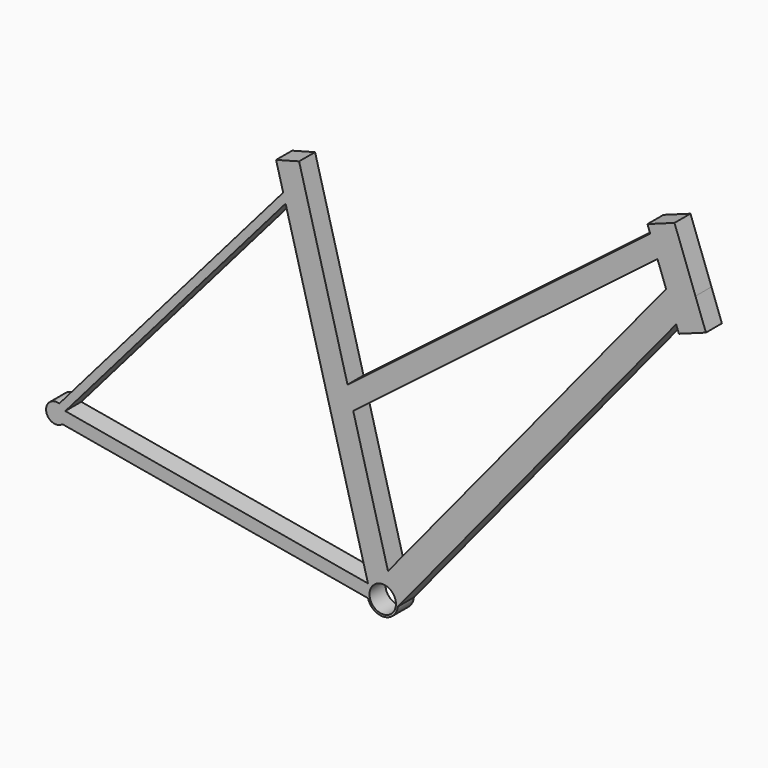
from build123d import *

# Parameters (mm, degrees)
F1_R     = 16.55
F0_DEPTH = 25


with BuildPart() as f0:
    # F1 (on Front) → F0 (new body)
    with BuildSketch(Plane.XZ):
        with BuildLine():
            ThreePointArc((18.9471511403, -1.9768570177), (19.0242704094, -0.9897653202), (19.05, 0))
            ThreePointArc((19.05, 0), (17.0081092666, 8.5806013294), (11.3201607165, 15.3217643028))
            ThreePointArc((11.3201607165, 15.3217643028), (3.1862146863, 18.7816542395), (-5.6337146577, 18.1979053508))
            ThreePointArc((-5.6337146577, 18.1979053508), (-12.7048225923, 14.1947167248), (-17.4644289069, 7.6089567588))
            ThreePointArc((-17.4644289069, 7.6089567588), (-18.9951016681, 1.4452033137), (-18.4145629505, -4.8791773224))
            ThreePointArc((-18.4145629505, -4.8791773224), (1.4753909085, -18.9927807776), (18.9471511403, -1.9768570177))
        make_face()
        Circle(F1_R, mode=Mode.SUBTRACT)
        with BuildLine():
            ThreePointArc((11.3201607165, 15.3217643028), (17.0081092666, 8.5806013294), (19.05, 0))
            ThreePointArc((19.05, 0), (19.0242704094, -0.9897653202), (18.9471511403, -1.9768570177))
            Line((18.9471511403, -1.9768570177), (367.068516355, 422.1730984288))
            Line((367.068516355, 422.1730984288), (358.5591705204, 445.5523339637))
            Line((358.5591705204, 445.5523339637), (354.4296862364, 456.8979987878))
            Line((354.4296862364, 456.8979987878), (197.6336692676, 265.8582343353))
            Line((197.6336692676, 265.8582343353), (68.718206586, 108.788047853))
            Line((68.718206586, 108.788047853), (6.5665120874, 33.0626225082))
            Line((6.5665120874, 33.0626225082), (11.3201607165, 15.3217643028))
        make_face()
        with BuildLine():
            ThreePointArc((-5.6337146577, 18.1979053508), (3.1862146863, 18.7816542395), (11.3201607165, 15.3217643028))
            Line((11.3201607165, 15.3217643028), (6.5665120874, 33.0626225082))
            Line((6.5665120874, 33.0626225082), (-36.9494436056, 195.4663800944))
            Line((-36.9494436056, 195.4663800944), (-44.0597309982, 222.0023338999))
            Line((-44.0597309982, 222.0023338999), (-104.6644659355, 448.182283865))
            Line((-104.6644659355, 448.182283865), (-133.4490555589, 440.4694763209))
            Line((-133.4490555589, 440.4694763209), (-124.5620482674, 407.302713582))
            Line((-124.5620482674, 407.302713582), (-121.5848978652, 396.1918370193))
            Line((-121.5848978652, 396.1918370193), (-18.4742653371, 11.3777176238))
            Line((-18.4742653371, 11.3777176238), (-17.4644289069, 7.6089567588))
            ThreePointArc((-17.4644289069, 7.6089567588), (-12.7048225923, 14.1947167248), (-5.6337146577, 18.1979053508))
        make_face()
        with BuildLine():
            Line((-72.3879589454, 4.6290750499), (-18.4145629505, -4.8791773224))
            ThreePointArc((-18.4145629505, -4.8791773224), (-18.9951016681, 1.4452033137), (-17.4644289069, 7.6089567588))
            Line((-17.4644289069, 7.6089567588), (-18.4742653371, 11.3777176238))
            Line((-18.4742653371, 11.3777176238), (-69.612055331, 20.3864339378))
            ThreePointArc((-69.612055331, 20.3864339378), (-70.9081149957, 12.4915662651), (-72.3879589454, 4.6290750499))
        make_face()
        Polygon((358.5591705204, 445.5523339637), (367.068516355, 422.1730984288), (370.4887177882, 412.7761722209), (387.4031849624, 418.9325348008), (404.3176521365, 425.0888973806), (391.2308402699, 461.0446174767), (364.9853356541, 533.153548771), (331.1564013058, 520.8408236113), (334.576602739, 511.4438974034), (343.6802788522, 486.4317528486), (354.4296862364, 456.8979987878), align=None)
        Polygon((-44.0597309982, 222.0023338999), (-36.9494436056, 195.4663800944), (128.9154626816, 322.2587492585), (343.6802788522, 486.4317528486), (334.576602739, 511.4438974034), align=None)
        with BuildLine():
            Line((-103.9121348451, 10.1825484742), (-72.3879589454, 4.6290750499))
            ThreePointArc((-72.3879589454, 4.6290750499), (-70.9081149957, 12.4915662651), (-69.612055331, 20.3864339378))
            Line((-69.612055331, 20.3864339378), (-101.1362312306, 25.9399073622))
            ThreePointArc((-101.1362312306, 25.9399073622), (-102.4228327716, 18.043373494), (-103.9121348451, 10.1825484742))
        make_face()
        with BuildLine():
            Line((-124.5620482674, 407.302713582), (-187.7531740158, 334.3521096451))
            ThreePointArc((-187.7531740158, 334.3521096451), (-184.1317567279, 331.2589177075), (-180.5536370153, 328.1157411523))
            Line((-180.5536370153, 328.1157411523), (-121.5848978652, 396.1918370193))
            Line((-121.5848978652, 396.1918370193), (-124.5620482674, 407.302713582))
        make_face()
        with BuildLine():
            ThreePointArc((-180.5536370153, 328.1157411523), (-184.1317567279, 331.2589177075), (-187.7531740158, 334.3521096451))
            Line((-187.7531740158, 334.3521096451), (-208.7069809814, 310.1621169077))
            ThreePointArc((-208.7069809814, 310.1621169077), (-205.0833359165, 307.0714968135), (-201.5074439809, 303.9257484149))
            Line((-201.5074439809, 303.9257484149), (-180.5536370153, 328.1157411523))
        make_face()
        with BuildLine():
            Line((-400.6354173431, 62.4549653328), (-103.9121348451, 10.1825484742))
            ThreePointArc((-103.9121348451, 10.1825484742), (-102.4228327716, 18.043373494), (-101.1362312306, 25.9399073622))
            Line((-101.1362312306, 25.9399073622), (-397.1350282031, 78.084694838))
            Line((-397.1350282031, 78.084694838), (-201.5074439809, 303.9257484149))
            ThreePointArc((-201.5074439809, 303.9257484149), (-205.0833359165, 307.0714968135), (-208.7069809814, 310.1621169077))
            Line((-208.7069809814, 310.1621169077), (-404.7393478146, 83.8537645513))
            ThreePointArc((-404.7393478146, 83.8537645513), (-398.5615625862, 79.3027613179), (-396.2064961559, 72))
            ThreePointArc((-396.2064961559, 72), (-397.3676583592, 66.7387494433), (-400.6354173431, 62.4549653328))
        make_face()
        with BuildLine():
            ThreePointArc((-404.7393478146, 83.8537645513), (-420.9827692162, 69.6456169071), (-400.6354173431, 62.4549653328))
            ThreePointArc((-400.6354173431, 62.4549653328), (-397.3676583592, 66.7387494433), (-396.2064961559, 72))
            ThreePointArc((-396.2064961559, 72), (-398.5615625862, 79.3027613179), (-404.7393478146, 83.8537645513))
        make_face()
    extrude(amount=F0_DEPTH)


solid = f0.part
